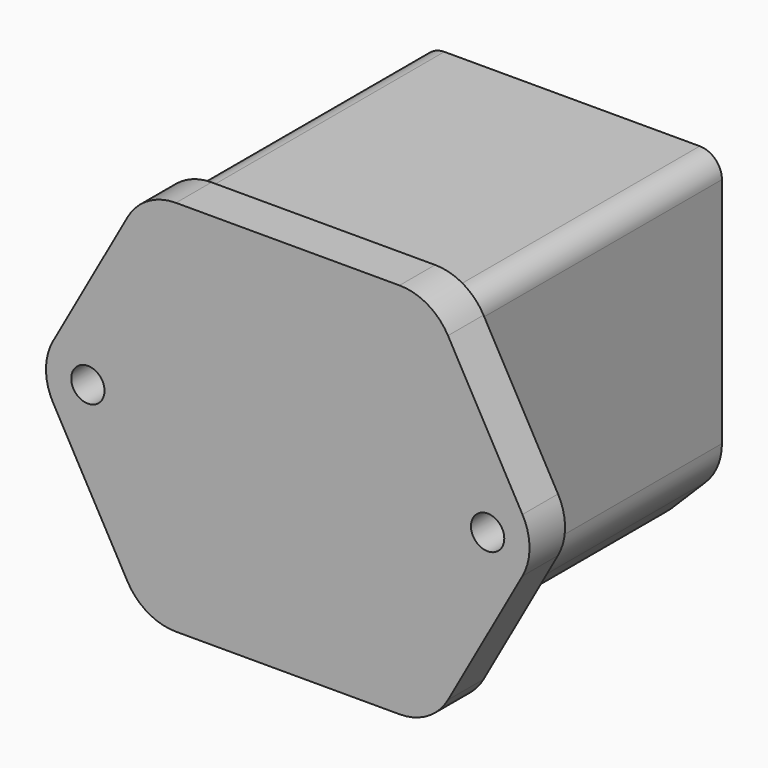
from build123d import *

# Parameters (mm, degrees)
F1_DEPTH = 4
F2_W     = 27
F2_H     = 31
F3_DEPTH = 28
F4_R     = 2
F5_R     = 5
F6_R     = 1.5
F7_DEPTH = 25
F8_SIZE  = 6
F9_R     = 5
F10_R    = 5


with BuildPart() as f1:
    # F0 (on Front) → F1 (new body)
    with BuildSketch(Plane.XZ):
        Polygon((-13, -17), (13, -17), (22.5, 0), (13, 17), (-13, 17), (-22.5, 0), align=None)
    extrude(amount=F1_DEPTH)

    # F2 (on face) → F3 (join)
    with BuildSketch(Plane(origin=(0, 0, 0), x_dir=(-1, 0, 0), z_dir=(0, 1, 0))):
        Rectangle(F2_W, F2_H)
    extrude(amount=F3_DEPTH)

    # F4
    f4_edges = [f1.edges().sort_by_distance(p)[0] for p in [
        (-13.5, 14, 15.5),
        (13.5, 14, 15.5),
    ]]
    fillet(f4_edges, radius=F4_R)

    # F5
    f5_edges = [f1.edges().sort_by_distance(p)[0] for p in [
        (-22.5, -2, 0),
        (22.5, -2, 0),
    ]]
    fillet(f5_edges, radius=F5_R)

    # F6 (on face) → F7 (cut)
    with BuildSketch(Plane.XZ.offset(4)):
        with Locations((-18, 0)):
            Circle(F6_R)
        with Locations((18, 0)):
            Circle(F6_R)
    extrude(amount=-F7_DEPTH, mode=Mode.SUBTRACT)

    # F8
    f8_edges = [f1.edges().sort_by_distance(p)[0] for p in [
        (13.5, 14, -15.5),
        (-13.5, 14, -15.5),
    ]]
    chamfer(f8_edges, length=F8_SIZE)

    # F9
    f9_edges = [f1.edges().sort_by_distance(p)[0] for p in [
        (13, -2, 17),
        (-13, -2, 17),
        (13, -2, -17),
        (-13, -2, -17),
    ]]
    fillet(f9_edges, radius=F9_R)

    # F10
    f10_edges = [f1.edges().sort_by_distance(p)[0] for p in [
        (-13.5, 14, -9.5),
        (-7.5, 14, -15.5),
        (7.5, 14, -15.5),
        (13.5, 14, -9.5),
    ]]
    fillet(f10_edges, radius=F10_R)


solid = f1.part
